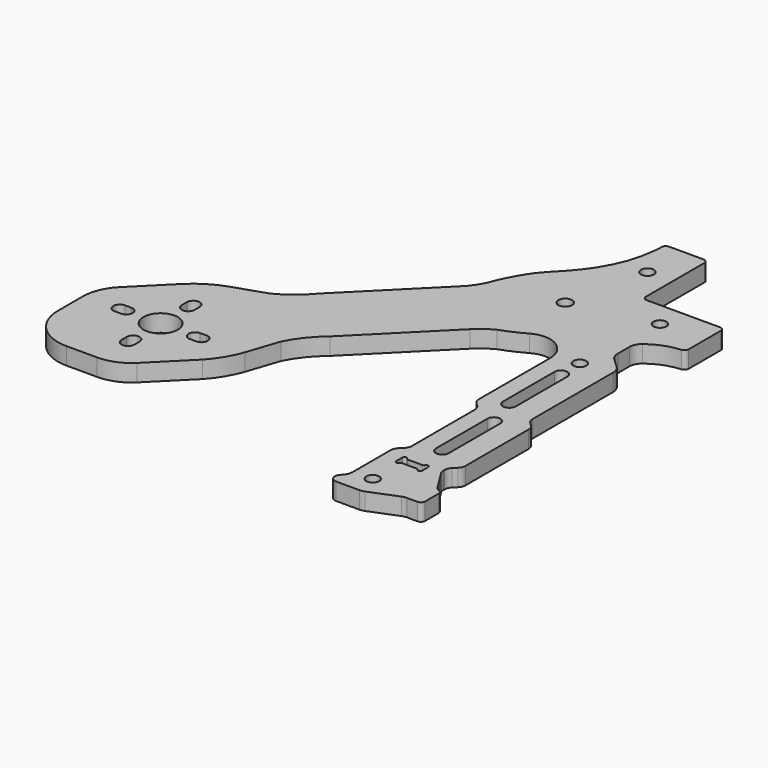
from build123d import *

# Parameters (mm, degrees)
F0_R     = 4
F0_R_2   = 1.5
F0_R_3   = 1.6
F1_DEPTH = 4


# Not quite as in the source:
# - ends of sketch curves that miss each other by under 0.0002 mm in the source are joined


with BuildPart() as f1:
    # F0 (on Top) → F1 (new body)
    with BuildSketch(Plane.XY):
        with BuildLine():
            ThreePointArc((30.9978440056, -52.3819660063), (30.5965854602, -54.0352331312), (31.997844, -55))
            Line((31.997844, -55), (37.420097, -55))
            ThreePointArc((37.420097, -55), (37.9874195635, -54.9458691602), (38.5342690291, -54.7854300727))
            Line((38.5342690291, -54.7854300727), (44.961419, -52.21457))
            ThreePointArc((44.961419, -52.21457), (45.5082684365, -52.0541308398), (46.075591, -52))
            Line((46.075591, -52), (48.497844, -52))
            ThreePointArc((48.497844, -52), (49.2049507812, -51.7071067812), (49.497844, -51))
            Line((49.497844, -51), (49.497844, -47.054858))
            ThreePointArc((49.497844, -47.054858), (49.3143367471, -46.477502309), (48.8311648121, -46.1120445316))
            ThreePointArc((48.8311648121, -46.1120445316), (48.2464480359, -45.7865652768), (47.8018474974, -45.2864046891))
            Line((47.8018474974, -45.2864046891), (44.801847, -40.486405))
            ThreePointArc((44.801847, -40.486405), (44.5753463762, -39.9777725676), (44.497844, -39.426408))
            Line((44.497844, -39.426408), (44.497844, -39.145707))
            ThreePointArc((44.497844, -39.145707), (44.650084935, -38.3803401353), (45.0836304376, -37.7314934376))
            Line((45.0836304376, -37.7314934376), (45.912058, -36.903066))
            ThreePointArc((45.912058, -36.903066), (46.3456032003, -36.2542195381), (46.497844, -35.488853))
            Line((46.497844, -35.488853), (46.497844, -17.145707))
            ThreePointArc((46.497844, -17.145707), (46.345603065, -16.3803401353), (45.9120575624, -15.7314934376))
            Line((45.9120575624, -15.7314934376), (45.08363, -14.903066))
            ThreePointArc((45.08363, -14.903066), (44.6500847997, -14.2542195381), (44.497844, -13.488853))
            Line((44.497844, -13.488853), (44.497844, 9.963987))
            ThreePointArc((44.497844, 9.963987), (44.2491834617, 11.1598679166), (43.5444232222, 12.1575032382))
            Line((43.5444232222, 12.1575032382), (41.451265, 14.110446))
            ThreePointArc((41.451265, 14.110446), (40.7465046743, 15.1080817706), (40.497844, 16.303963))
            Line((40.497844, 16.303963), (40.497844, 19.657184))
            ThreePointArc((40.497844, 19.657184), (40.8005276064, 20.970380205), (41.6475001819, 22.0185877679))
            ThreePointArc((41.6475001819, 22.0185877679), (44.9097367641, 23.8722057946), (48.5706879935, 24.6941080891))
            ThreePointArc((48.5706879935, 24.6941080891), (49.2302523646, 25.0105853837), (49.497844, 25.691451))
            Line((49.497844, 25.691451), (49.497844, 35))
            ThreePointArc((49.497844, 35), (49.2049507812, 35.7071067812), (48.497844, 36))
            Line((48.497844, 36), (31.497844, 36))
            ThreePointArc((31.497844, 36), (30.7907372188, 36.2928932188), (30.497844, 37))
            Line((30.497844, 37), (30.497844, 54))
            ThreePointArc((30.497844, 54), (30.2049507812, 54.7071067812), (29.497844, 55))
            Line((29.497844, 55), (21.513528, 55))
            ThreePointArc((21.513528, 55), (20.8178624993, 54.7183658616), (20.5140433064, 54.0320990223))
            ThreePointArc((20.5140433064, 54.0320990223), (20.4696724232, 53.1001685974), (20.3964907955, 52.1700570193))
            ThreePointArc((20.3964907955, 52.1700570193), (19.0508324444, 46.0085107955), (16.2674640132, 40.3491549914))
            ThreePointArc((16.2674640132, 40.3491549914), (14.1457607442, 37.4387671742), (11.7343381171, 34.7635058829))
            ThreePointArc((11.7343381171, 34.7635058829), (10.1184707238, 33.0449295675), (8.6114374257, 31.2301616681))
            ThreePointArc((8.6114374257, 31.2301616681), (6.2460068014, 27.2541578949), (4.4197862212, 23.0034182758))
            ThreePointArc((4.4197862212, 23.0034182758), (3.0950438794, 20.8390250787), (1.4145833361, 18.9375536462))
            Line((1.4145833361, 18.9375536462), (-16.61664, 0.906331))
            ThreePointArc((-16.61664, 0.906331), (-19.8548943434, -2.2936956172), (-23.6877079435, -4.7505231125))
            Line((-23.6877079435, -4.7505231125), (-31.112329, -7.225397))
            ThreePointArc((-31.112329, -7.225397), (-34.8708228196, -8.9751171402), (-38.1833968947, -11.4680371131))
            Line((-38.1833968947, -11.4680371131), (-46.668678, -19.953319))
            ThreePointArc((-46.668678, -19.953319), (-48.7861533831, -23.2075482546), (-49.4971053712, -27.0243870045))
            Line((-49.4971053712, -27.0243870045), (-49.497105, -34.095454))
            ThreePointArc((-49.497105, -34.095454), (-46.5976100448, -41.0954540448), (-39.59761, -43.994949))
            Line((-39.59761, -43.994949), (-32.526543, -43.994949))
            ThreePointArc((-32.526543, -43.994949), (-28.7097042546, -43.2839973831), (-25.455474662, -41.1665223463))
            Line((-25.455474662, -41.1665223463), (-16.970193, -32.681241))
            ThreePointArc((-16.970193, -32.681241), (-14.4772731402, -29.3686668196), (-12.7275523092, -25.6101732374))
            Line((-12.7275523092, -25.6101732374), (-10.252679, -18.185552))
            ThreePointArc((-10.252679, -18.185552), (-7.7958516172, -14.3527383434), (-4.5958249273, -11.1144840887))
            Line((-4.5958249273, -11.1144840887), (13.497844, 7))
            ThreePointArc((13.497844, 7), (15.3717346163, 8.6360982299), (17.5012621548, 9.9219426844))
            ThreePointArc((17.5012621548, 9.9219426844), (20.331733184, 11.063946628), (23.0532060982, 12.4457298257))
            ThreePointArc((23.0532060982, 12.4457298257), (29.0253982797, 12.3981522415), (31.997844, 7.218006))
            Line((31.997844, 7.218006), (31.997844, -13.488853))
            ThreePointArc((31.997844, -13.488853), (32.1500847997, -14.2542195381), (32.5836299376, -14.9030660624))
            Line((32.5836299376, -14.9030660624), (33.412058, -15.731493))
            ThreePointArc((33.412058, -15.731493), (33.845603065, -16.3803401353), (33.997844, -17.145707))
            Line((33.997844, -17.145707), (33.997844, -35.488853))
            ThreePointArc((33.997844, -35.488853), (33.8456032003, -36.2542195381), (33.4120580624, -36.9030660624))
            Line((33.4120580624, -36.9030660624), (32.58363, -37.731493))
            ThreePointArc((32.58363, -37.731493), (32.150084935, -38.3803401353), (31.997844, -39.145707))
            Line((31.997844, -39.145707), (31.997844, -50.145898))
            ThreePointArc((31.997844, -50.145898), (31.7364567845, -51.3706428782), (30.9978440056, -52.3819660063))
        make_face()
        with BuildLine():
            ThreePointArc((-33.319436, -34.31728), (-31.819436, -32.81728), (-30.319436, -34.31728))
            Line((-30.319436, -34.31728), (-30.319436, -35.81728))
            ThreePointArc((-30.319436, -35.81728), (-31.819436, -37.31728), (-33.319436, -35.81728))
            Line((-33.319436, -35.81728), (-33.319436, -34.31728))
        make_face(mode=Mode.SUBTRACT)
        with BuildLine():
            ThreePointArc((-41.319436, -27.81728), (-42.819436, -26.31728), (-41.319436, -24.81728))
            Line((-41.319436, -24.81728), (-39.819436, -24.81728))
            ThreePointArc((-39.819436, -24.81728), (-38.319436, -26.31728), (-39.819436, -27.81728))
            Line((-39.819436, -27.81728), (-41.319436, -27.81728))
        make_face(mode=Mode.SUBTRACT)
        with Locations((-31.819436, -26.31728)):
            Circle(F0_R, mode=Mode.SUBTRACT)
        with BuildLine():
            ThreePointArc((-33.319436, -16.81728), (-31.819436, -15.31728), (-30.319436, -16.81728))
            Line((-30.319436, -16.81728), (-30.319436, -18.31728))
            ThreePointArc((-30.319436, -18.31728), (-31.819436, -19.81728), (-33.319436, -18.31728))
            Line((-33.319436, -18.31728), (-33.319436, -16.81728))
        make_face(mode=Mode.SUBTRACT)
        with BuildLine():
            ThreePointArc((-23.819436, -27.81728), (-25.319436, -26.31728), (-23.819436, -24.81728))
            Line((-23.819436, -24.81728), (-22.319436, -24.81728))
            ThreePointArc((-22.319436, -24.81728), (-20.819436, -26.31728), (-22.319436, -27.81728))
            Line((-22.319436, -27.81728), (-23.819436, -27.81728))
        make_face(mode=Mode.SUBTRACT)
        with Locations((36.497844, -50)):
            Circle(F0_R_2, mode=Mode.SUBTRACT)
        with BuildLine():
            Line((41.522844, -40.125), (41.522844, -41.875))
            ThreePointArc((41.522844, -41.875), (41.1522534506, -42.3579629324), (40.5898312236, -42.1249998709))
            ThreePointArc((40.5898312236, -42.1249998709), (40.406818848, -41.9419872104), (40.156819, -41.875))
            Line((40.156819, -41.875), (36.838869, -41.875))
            ThreePointArc((36.838869, -41.875), (36.588869152, -41.9419872104), (36.4058564736, -42.1249996961))
            ThreePointArc((36.4058564736, -42.1249996961), (35.8434345494, -42.3579629324), (35.472844, -41.875))
            Line((35.472844, -41.875), (35.472844, -40.125))
            ThreePointArc((35.472844, -40.125), (35.8434345494, -39.6420370676), (36.4058567764, -39.8750001291))
            ThreePointArc((36.4058567764, -39.8750001291), (36.588869152, -40.0580127896), (36.838869, -40.125))
            Line((36.838869, -40.125), (40.156819, -40.125))
            ThreePointArc((40.156819, -40.125), (40.406818848, -40.0580127896), (40.5898315264, -39.8750003039))
            ThreePointArc((40.5898315264, -39.8750003039), (41.1522534506, -39.6420370676), (41.522844, -40.125))
        make_face(mode=Mode.SUBTRACT)
        with BuildLine():
            Line((40.997844, -18.5), (40.997844, -33.5))
            ThreePointArc((40.997844, -33.5), (39.497844, -35), (37.997844, -33.5))
            Line((37.997844, -33.5), (37.997844, -18.5))
            ThreePointArc((37.997844, -18.5), (39.497844, -17), (40.997844, -18.5))
        make_face(mode=Mode.SUBTRACT)
        with BuildLine():
            Line((38.997844, 3.5), (38.997844, -11.5))
            ThreePointArc((38.997844, -11.5), (37.497844, -13), (35.997844, -11.5))
            Line((35.997844, -11.5), (35.997844, 3.5))
            ThreePointArc((35.997844, 3.5), (37.497844, 5), (38.997844, 3.5))
        make_face(mode=Mode.SUBTRACT)
        with Locations((20.497844, 26)):
            Circle(F0_R_3, mode=Mode.SUBTRACT)
        with Locations((37.497844, 9)):
            Circle(F0_R_2, mode=Mode.SUBTRACT)
        with Locations((24.673148, 44.716341)):
            Circle(F0_R_2, mode=Mode.SUBTRACT)
        with Locations((39.215118, 30.174371)):
            Circle(F0_R_2, mode=Mode.SUBTRACT)
    extrude(amount=F1_DEPTH)


solid = f1.part
